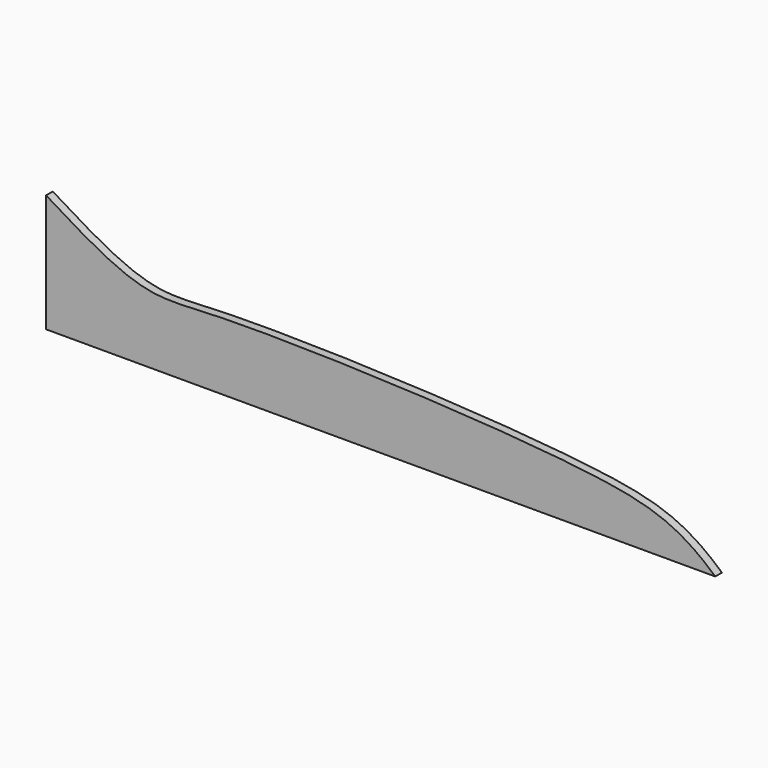
from build123d import *

# Parameters (mm, degrees)
F0_W     = 80
F0_H     = 15
F1_DEPTH = 10
F3_DEPTH = 80
F5_DEPTH = 1


# Not quite as in the source:
# - a feature names something its author has since deleted; it is built from what else it names


with BuildPart() as f1:
    # F0 (on Front) → F1 (new body)
    with BuildSketch(Plane.XZ):
        with Locations((40, 7.5)):
            Rectangle(F0_W, F0_H)
    extrude(amount=-F1_DEPTH)

    # F2 (on face) → F3 (cut, through all)
    with BuildSketch(Plane.YZ.offset(80)):
        Polygon((0, 0), (3.8646364119, 0), (3.8646364119, 14.1026135534), (4.8646364119, 14.1026135534), (4.8646364119, 0), (10, 0), (10, 15), (0, 15), align=None)
    extrude(amount=-F3_DEPTH, mode=Mode.SUBTRACT)

    # F4 (on face) → F5 (cut, through all)
    with BuildSketch(Plane.XZ.offset(-3.8646364119)):
        with BuildLine():
            Line((80, 14.1026135534), (0, 14.1026135534))
            add(Edge.make_bspline(
                [(0, 14.1026135534), (11.4500320441, 6.9391493751), (14.6371912, 8.9491259409), (66.2321012405, 7.0001102922), (75.6593212739, 3.937227071), (80, 0)],
                knots=[0, 0, 0, 0, 0.2965600092, 0.7356986957, 1, 1, 1, 1], degree=3))
            Line((80, 0), (80, 14.1026135534))
        make_face()
    extrude(amount=-F5_DEPTH, mode=Mode.SUBTRACT)


solid = f1.part
